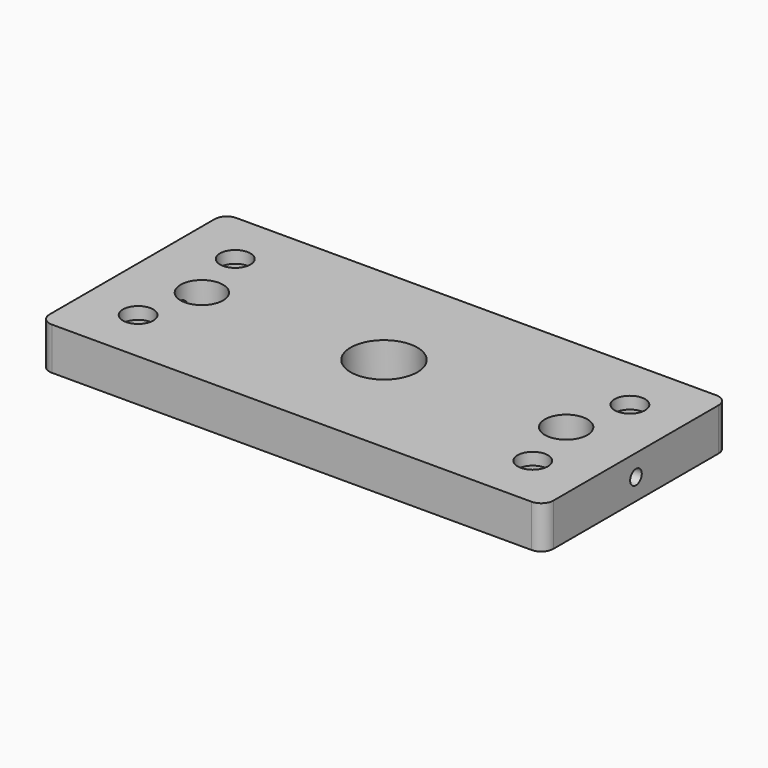
from build123d import *

# Parameters (mm, degrees)
F0_W      = 65
F0_H      = 20
F1_DEPTH  = 7
F2_D      = 5
F3_R      = 3.5
F4_DEPTH  = 25
F6_D      = 2.4
F6_DEPTH  = 11.8
F6_TIP    = 0.7210327428
F8_R      = 5.5
F9_DEPTH  = 25
F10_R     = 3.5
F11_DEPTH = 5


# Not quite as in the source:
# - a pattern or mirror of a feature is missing from the dataset's text; its kind, count and spacing are read off the source's solid


with BuildPart() as f1:
    # F0 (on Top) → F1 (new body)
    with BuildSketch(Plane.XY):
        with BuildLine():
            ThreePointArc((9, 27), (8.4142135624, 28.4142135624), (7, 29))
            Line((7, 29), (-72, 29))
            ThreePointArc((-72, 29), (-73.4142135624, 28.4142135624), (-74, 27))
            Line((-74, 27), (-74, -7))
            ThreePointArc((-74, -7), (-73.4142135624, -8.4142135624), (-72, -9))
            Line((-72, -9), (7, -9))
            ThreePointArc((7, -9), (8.4142135624, -8.4142135624), (9, -7))
            Line((9, -7), (9, 27))
        make_face()
        with Locations((-32.5, 10)):
            Rectangle(F0_W, F0_H, mode=Mode.SUBTRACT)
        with Locations((-32.5, 10)):
            Rectangle(F0_W, F0_H)
    extrude(amount=F1_DEPTH)

    # F2 (through all)
    with Locations(Plane(origin=(0, 0, 0), x_dir=(1, 0, 0), z_dir=(0, 0, -1))):
        with Locations((-65, -20), (-65, 0), (0, 0), (0, -20)):
            Hole(F2_D / 2)

    # F3 (on face) → F4 (cut)
    with BuildSketch(Plane.XY.offset(7)):
        with Locations((-62.5, 10)):
            Circle(F3_R)
        with Locations((-2.5, 10)):
            Circle(F3_R)
    extrude(amount=-F4_DEPTH, mode=Mode.SUBTRACT)

    # F6
    with Locations(Plane.YZ.offset(9)):
        with Locations((10, 3.5)):
            f6 = Hole(F6_D / 2, depth=F6_DEPTH)
            with Locations((0, 0, -(F6_DEPTH + F6_TIP / 2))):  # 118° drill point
                Cone(0, F6_D / 2, F6_TIP, mode=Mode.SUBTRACT)

    # F6_copies: F6 across plane
    add(f6.mirror(Plane(origin=(-32.500003, -1e-06, 0), x_dir=(0, 0, -1), z_dir=(-1, 0, 0))), mode=Mode.SUBTRACT)

    # F8 (on face) → F9 (cut)
    with BuildSketch(Plane.XY.offset(7)):
        with Locations((-32.5, 10)):
            Circle(F8_R)
    extrude(amount=-F9_DEPTH, mode=Mode.SUBTRACT)

    # F10 (on face) → F11 (cut)
    with BuildSketch(Plane.XY):
        Circle(F10_R)
        with Locations((-65, 0)):
            Circle(F10_R)
        with Locations((0, 20)):
            Circle(F10_R)
        with Locations((-65, 20)):
            Circle(F10_R)
    extrude(amount=F11_DEPTH, mode=Mode.SUBTRACT)


solid = f1.part
